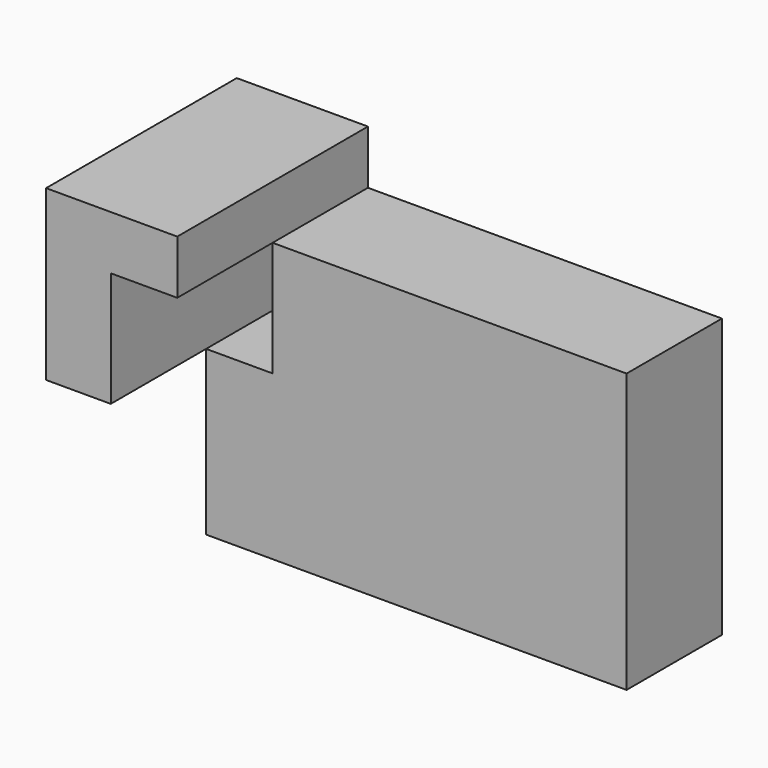
from build123d import *

# Parameters (mm, degrees)
F1_DEPTH = 25
F2_DEPTH = 25


with BuildPart() as f1:
    # F0 (on Front) → F1 (new body)
    with BuildSketch(Plane.XZ):
        Polygon((-37.5076346099, 27.2354409099), (-23.560071364, 27.2354409099), (-23.560071364, 38.5442748666), (-51.0782338679, 38.5442748666), (-51.0782338679, 3.1099293847), (-37.5076346099, 3.1099293847), align=None)
    extrude(amount=F1_DEPTH)

    # F2 (add): a face of the model
    f2_faces = [f1.faces().sort_by_distance(p)[0] for p in [
        (-40.8944956817, -25, 23.8065550076),
    ]]


with BuildPart() as f1b:
    # F0 (on Front) → F1, piece 2 (new body)
    with BuildSketch(Plane.XZ):
        Polygon((-12.6281967387, 27.2354409099), (-12.816679664, 27.2354409099), (-23.560071364, 27.2354409099), (-23.560071364, 3.1099293847), (-37.5076346099, 3.1099293847), (-37.5076346099, -31.1935339123), (50.7012717426, -31.1935339123), (50.7012717426, 27.2354409099), align=None)
    extrude(amount=F1_DEPTH)


with BuildPart() as f1_1:
    add(f1.part)

    add(f1b.part)  # F2 merges F1b
    extrude(f2_faces, amount=F2_DEPTH)


solid = f1_1.part
